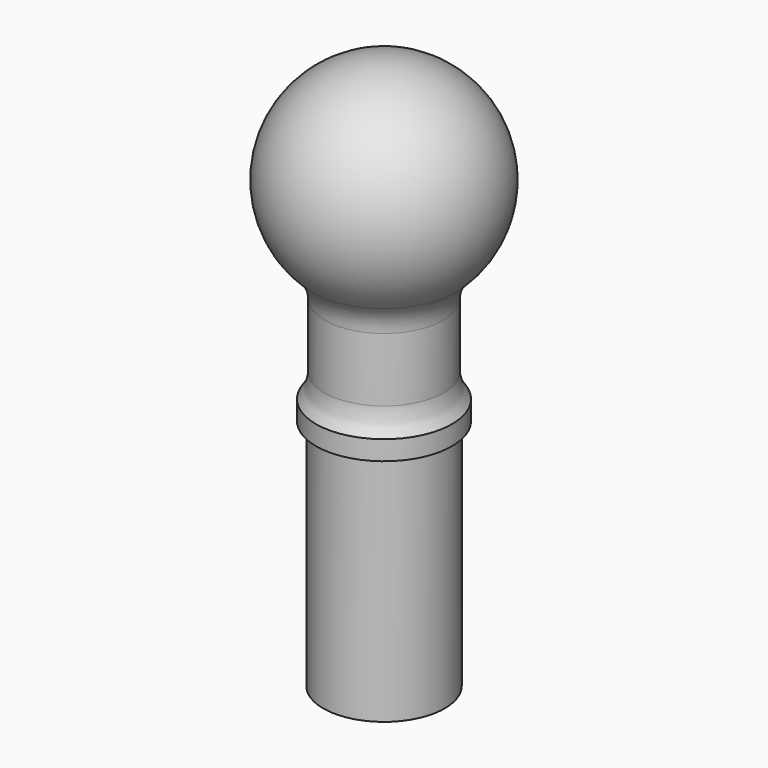
from build123d import *


# Not quite as in the source:
# - a fillet or chamfer that OpenCascade refuses, or shapes differently, is made with other operations: its cross-section is extruded or revolved along the edge and cut away or added


with BuildPart() as f1:
    # F0 (on Front) → F1 (revolve)
    with BuildSketch(Plane.XZ):
        with BuildLine():
            Line((-3.125, 0), (0, 0))
            Line((0, 0), (0, 28.3))
            ThreePointArc((0, 28.3), (-5.1322292743, 24.5221373378), (-3.05, 18.4991526235))
            Line((-3.05, 18.4991526235), (-3.05, 13))
            Line((-3.05, 13), (-3.5, 13))
            Line((-3.5, 13), (-3.5, 12))
            Line((-3.5, 12), (-3.125, 12))
            Line((-3.125, 12), (-3.125, 0))
        make_face()
    revolve(axis=Axis((0, 0, 7.9435938051), (0, 0, -1)))

    # F2: fillet of radius 2 on 2 edges, made by hand

    # F2_s1 → F2_t2 (revolve)
    with BuildSketch(Plane.XZ):
        with BuildLine():
            ThreePointArc((-3.6805084746, 19.0077966138), (-3.214382522, 18.3442782008), (-3.05, 17.5502325632))
            Line((-3.05, 17.5502325632), (-3.01, 17.5502325632))
            Line((-3.01, 17.5502325632), (-3.01, 18.4991526235))
            Line((-3.01, 18.4991526235), (-3.0273023256, 18.5320891621))
            ThreePointArc((-3.0273023256, 18.5320891621), (-3.3497353131, 18.7727116752), (-3.6531186441, 19.0369478948))
            Line((-3.6531186441, 19.0369478948), (-3.6805084746, 19.0077966138))
        make_face()
    revolve(axis=Axis((0, 0, 18.4991526235), (0, 0, -1)))

    # F2_s3 → F2_t4 (revolve)
    with BuildSketch(Plane.XZ):
        with BuildLine():
            ThreePointArc((-3.05, 14.263922466), (-3.1658556319, 13.5931020727), (-3.5, 13))
            Line((-3.5, 13), (-3.469, 12.9747215507))
            ThreePointArc((-3.469, 12.9747215507), (-3.275, 12.96), (-3.05, 12.96))
            Line((-3.05, 12.96), (-3.01, 13))
            Line((-3.01, 13), (-3.01, 14.263922466))
            Line((-3.01, 14.263922466), (-3.05, 14.263922466))
        make_face()
    revolve(axis=Axis((0, 0, 13), (0, 0, -1)))


solid = f1.part
